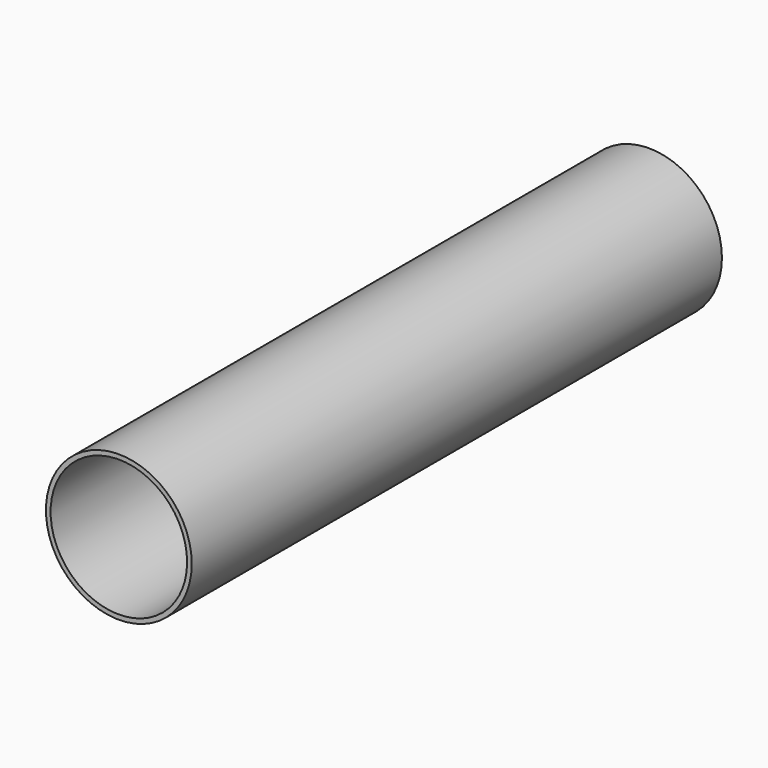
from build123d import *

# Parameters (mm, degrees)
F2_R     = 16.5
F2_R_2   = 15.45
F3_DEPTH = 150


# Not quite as in the source:
# - the program builds the solid bodies; features that only make, move or delete a surface that nothing else refers to are left out


with BuildPart() as f3:
    # F2 (on Front) → F3 (new body)
    with BuildSketch(Plane.XZ):
        with Locations((-46.8991808593, 0)):
            Circle(F2_R)
        with Locations((-46.8991808593, 0)):
            Circle(F2_R_2, mode=Mode.SUBTRACT)
    extrude(amount=-F3_DEPTH)


solid = f3.part
